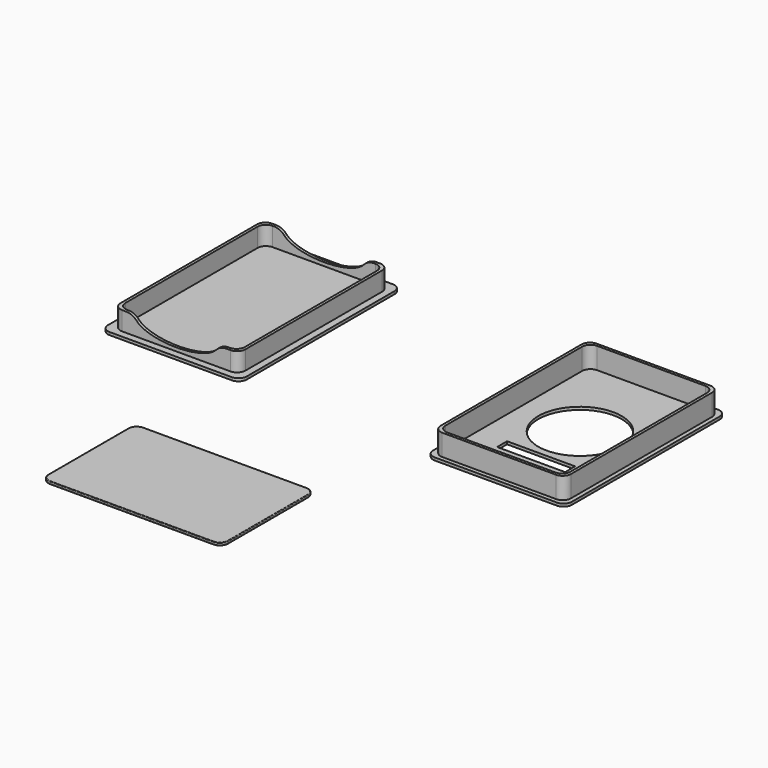
from build123d import *

# Parameters (mm, degrees)
F0_W        = 64.75
F0_H        = 42
F1_DEPTH    = 1
F2_R        = 3
F3_R        = 0.2
F0_W_2      = 50
F0_H_2      = 72.5
F0_W_3      = 45
F0_H_3      = 67.5
F0_W_4      = 43
F0_H_4      = 65.5
F4_DEPTH    = 1
F5_DEPTH    = 7.75
F6_R        = 3
F8_DEPTH    = 70.001
F9_T1_DEPTH = 1
F9_T3_DEPTH = 1
F0_W_5      = 47
F0_H_5      = 69.5
F0_W_6      = 24.5
F0_H_6      = 4.5
F0_R        = 15
F10_DEPTH   = 1
F11_DEPTH   = 8.7
F12_R       = 3


# Not quite as in the source:
# - a fillet or chamfer that OpenCascade refuses, or shapes differently, is made with other operations: its cross-section is extruded or revolved along the edge and cut away or added


with BuildPart() as f1:
    # F0 (on Top) → F1 (new body)
    with BuildSketch(Plane.XY):
        with Locations((-12.0692265069, -60.4423025408)):
            Rectangle(F0_W, F0_H)
    extrude(amount=F1_DEPTH)

    # F2
    f2_edges = [f1.edges().sort_by_distance(p)[0] for p in [
        (-44.444227, -39.442303, 0.5),
        (-44.444227, -81.442303, 0.5),
        (20.305773, -81.442303, 0.5),
        (20.305773, -39.442303, 0.5),
    ]]
    fillet(f2_edges, radius=F2_R)

    # F3
    f3_edges = [f1.edges().sort_by_distance(p)[0] for p in [
        (-12.069227, -39.442303, 1),
        (19.427094, -40.320982, 1),
        (-43.565547, -40.320982, 1),
        (20.305773, -60.442303, 1),
        (-44.444227, -60.442303, 1),
        (19.427094, -80.563623, 1),
        (-43.565547, -80.563623, 1),
        (-12.069227, -81.442303, 1),
        (-12.069227, -39.442303, 0),
        (19.427094, -40.320982, 0),
        (-43.565547, -40.320982, 0),
        (20.305773, -60.442303, 0),
        (-44.444227, -60.442303, 0),
        (19.427094, -80.563623, 0),
        (-43.565547, -80.563623, 0),
        (-12.069227, -81.442303, 0),
    ]]
    fillet(f3_edges, radius=F3_R)


with BuildPart() as f4:
    # F0 (on Top) → F4 (new body)
    with BuildSketch(Plane.XY):
        with Locations((-63.1516585421, 36.25)):
            Rectangle(F0_W_2, F0_H_2)
        with Locations((-63.1516585421, 36.25)):
            Rectangle(F0_W_3, F0_H_3, mode=Mode.SUBTRACT)
        with Locations((-63.1516585421, 36.25)):
            Rectangle(F0_W_3, F0_H_3)
        with Locations((-63.1516585421, 36.25)):
            Rectangle(F0_W_4, F0_H_4, mode=Mode.SUBTRACT)
        with Locations((-63.1516585421, 36.25)):
            Rectangle(F0_W_4, F0_H_4)
    extrude(amount=F4_DEPTH)

    # F0 (on Top) → F5 (join)
    with BuildSketch(Plane.XY):
        with Locations((-63.1516585421, 36.25)):
            Rectangle(F0_W_3, F0_H_3)
        with Locations((-63.1516585421, 36.25)):
            Rectangle(F0_W_4, F0_H_4, mode=Mode.SUBTRACT)
    extrude(amount=F5_DEPTH)

    # F6
    f6_edges = [f4.edges().sort_by_distance(p)[0] for p in [
        (-85.651659, 2.5, 4.375),
        (-40.651659, 2.5, 4.375),
        (-85.651659, 70, 4.375),
        (-40.651659, 70, 4.375),
        (-88.151659, 72.5, 0.5),
        (-38.151659, 72.5, 0.5),
        (-38.151659, 0, 0.5),
        (-88.151659, 0, 0.5),
        (-41.651659, 3.5, 4.375),
        (-84.651659, 3.5, 4.375),
        (-84.651659, 69, 4.375),
        (-41.651659, 69, 4.375),
    ]]
    fillet(f6_edges, radius=F6_R)

    # F7 (on face) → F8 (cut, through all)
    with BuildSketch(Plane.XZ.offset(-2.5)):
        with BuildLine():
            add(Edge.make_bspline(
                [(-48.1516585421, 7.75), (-48.1516585421, 17.2762794416), (-70.6516585421, 12.5131397208), (-93.1516585421, 7.75), (-70.6516585421, 2.9868602792), (-48.1516585421, -1.7762794416), (-48.1516585421, 7.75)],
                knots=[0, 0, 0, 2.0943951024, 2.0943951024, 4.1887902048, 4.1887902048, 6.2831853072, 6.2831853072, 6.2831853072], degree=2, weights=[1, 0.5, 1, 0.5, 1, 0.5, 1]))
        make_face()
    extrude(amount=-F8_DEPTH, mode=Mode.SUBTRACT)

    # F9: fillet of radius 5 on 4 edges, made by hand

    # F9_s2 → F9_t1 (cut)
    with BuildSketch(Plane.XZ.offset(-70)):
        with BuildLine():
            ThreePointArc((-81.1735034535, 7.75), (-79.116499703, 7.3072728216), (-77.423772539, 6.057494228))
            Line((-77.423772539, 6.057494228), (-77.3487779207, 6.1236441126))
            ThreePointArc((-77.3487779207, 6.1236441126), (-77.8507909347, 6.8746512138), (-78.0516585421, 7.75))
            Line((-78.0516585421, 7.75), (-78.1516585421, 7.85))
            Line((-78.1516585421, 7.85), (-81.1735034535, 7.85))
            Line((-81.1735034535, 7.85), (-81.1735034535, 7.75))
        make_face()
        with BuildLine():
            ThreePointArc((-45.1298136307, 7.75), (-47.1868173813, 7.3072728216), (-48.8795445453, 6.057494228))
            Line((-48.8795445453, 6.057494228), (-48.9545391636, 6.1236441126))
            ThreePointArc((-48.9545391636, 6.1236441126), (-48.4525261496, 6.8746512138), (-48.2516585421, 7.75))
            Line((-48.2516585421, 7.75), (-48.1516585421, 7.85))
            Line((-48.1516585421, 7.85), (-45.1298136307, 7.85))
            Line((-45.1298136307, 7.85), (-45.1298136307, 7.75))
        make_face()
    extrude(amount=F9_T1_DEPTH, mode=Mode.SUBTRACT)

    # F9_s4 → F9_t3 (cut)
    with BuildSketch(Plane.XZ.offset(-3.5)):
        with BuildLine():
            ThreePointArc((-81.1735034535, 7.75), (-79.116499703, 7.3072728216), (-77.423772539, 6.057494228))
            Line((-77.423772539, 6.057494228), (-77.3487779207, 6.1236441126))
            ThreePointArc((-77.3487779207, 6.1236441126), (-77.8507909347, 6.8746512138), (-78.0516585421, 7.75))
            Line((-78.0516585421, 7.75), (-78.1516585421, 7.85))
            Line((-78.1516585421, 7.85), (-81.1735034535, 7.85))
            Line((-81.1735034535, 7.85), (-81.1735034535, 7.75))
        make_face()
        with BuildLine():
            ThreePointArc((-45.1298136307, 7.75), (-47.1868173813, 7.3072728216), (-48.8795445453, 6.057494228))
            Line((-48.8795445453, 6.057494228), (-48.9545391636, 6.1236441126))
            ThreePointArc((-48.9545391636, 6.1236441126), (-48.4525261496, 6.8746512138), (-48.2516585421, 7.75))
            Line((-48.2516585421, 7.75), (-48.1516585421, 7.85))
            Line((-48.1516585421, 7.85), (-45.1298136307, 7.85))
            Line((-45.1298136307, 7.85), (-45.1298136307, 7.75))
        make_face()
    extrude(amount=F9_T3_DEPTH, mode=Mode.SUBTRACT)


with BuildPart() as f10:
    # F0 (on Top) → F10 (new body)
    with BuildSketch(Plane.XY):
        with Locations((55.9352879792, 33.75)):
            Rectangle(F0_W_2, F0_H_2)
        with Locations((55.9352879792, 33.75)):
            Rectangle(F0_W_5, F0_H_5, mode=Mode.SUBTRACT)
        with Locations((55.9352879792, 33.75)):
            Rectangle(F0_W_5, F0_H_5)
        with Locations((55.9352879792, 33.75)):
            Rectangle(F0_W_3, F0_H_3, mode=Mode.SUBTRACT)
        with Locations((55.9352879792, 33.75)):
            Rectangle(F0_W_3, F0_H_3)
        with Locations((55.9352879792, 15.65)):
            Rectangle(F0_W_6, F0_H_6, mode=Mode.SUBTRACT)
        with Locations((55.9352879792, 35.4)):
            Circle(F0_R, mode=Mode.SUBTRACT)
    extrude(amount=F10_DEPTH)

    # F0 (on Top) → F11 (join)
    with BuildSketch(Plane.XY):
        with Locations((55.9352879792, 33.75)):
            Rectangle(F0_W_5, F0_H_5)
        with Locations((55.9352879792, 33.75)):
            Rectangle(F0_W_3, F0_H_3, mode=Mode.SUBTRACT)
    extrude(amount=F11_DEPTH)

    # F12
    f12_edges = [f10.edges().sort_by_distance(p)[0] for p in [
        (80.935288, -2.5, 0.5),
        (79.435288, -1, 4.85),
        (78.435288, 0, 4.85),
        (30.935288, -2.5, 0.5),
        (32.435288, -1, 4.85),
        (33.435288, 0, 4.85),
        (33.435288, 67.5, 4.85),
        (78.435288, 67.5, 4.85),
        (32.435288, 68.5, 4.85),
        (30.935288, 70, 0.5),
        (80.935288, 70, 0.5),
        (79.435288, 68.5, 4.85),
    ]]
    fillet(f12_edges, radius=F12_R)


solid = Compound([f1.part, f4.part, f10.part])
